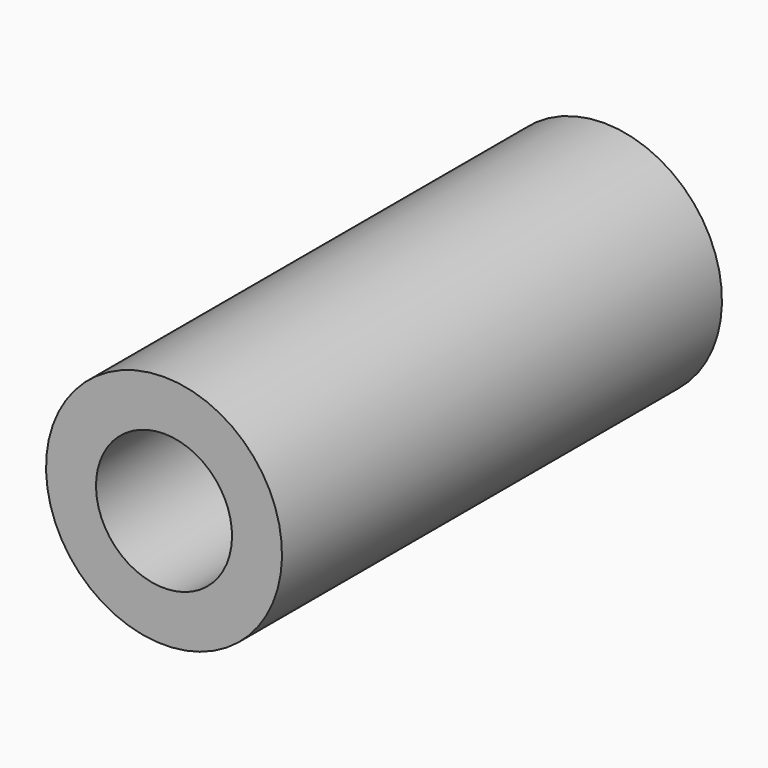
from build123d import *

# Parameters (mm, degrees)
F2_SIZE = 0.09999


# Not quite as in the source:
# - a fillet or chamfer is up to 0.001 mm smaller than in the source, because OpenCascade refuses the exact size


with BuildPart() as f1:
    # F0 (on Right) → F1 (revolve)
    with BuildSketch(Plane.YZ):
        Polygon((6.425, 3.3), (6.925, 2.8), (6.925, 3.3), align=None)
        with BuildLine():
            ThreePointArc((7.5617104388, 2.8), (8.3591026496, 4.0638625595), (9.425, 5.1112620751))
            Line((9.425, 5.1112620751), (9.425, 5.9))
            Line((9.425, 5.9), (-18.075, 5.9))
            Line((-18.075, 5.9), (-18.075, 3.4))
            Line((-18.075, 3.4), (-7.075, 3.4))
            Line((-7.075, 3.4), (-7.075, 3.3))
            Line((-7.075, 3.3), (-6.425, 3.3))
            Line((-6.425, 3.3), (6.425, 3.3))
            Line((6.425, 3.3), (6.925, 3.3))
            Line((6.925, 3.3), (6.925, 2.8))
            Line((6.925, 2.8), (7.5617104388, 2.8))
        make_face()
    revolve(axis=Axis((0, 1.503110514, 0), (0, 1, 0)))

    # F2 (size 0.1 in the source; OpenCascade refuses exactly that, so slightly less here)
    f2_edges = [f1.edges().sort_by_distance(p)[0] for p in [
        (0, -7.075, -3.4),
    ]]
    chamfer(f2_edges, length=F2_SIZE)


solid = f1.part
